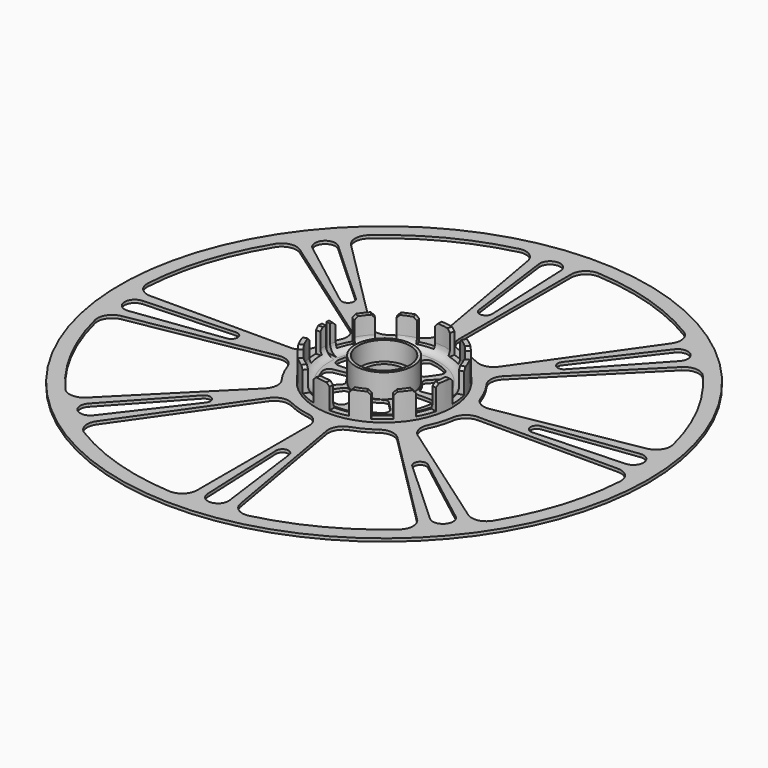
from build123d import *

# Parameters (mm, degrees)
F0_R      = 89
F0_R_2    = 6.5
F1_DEPTH  = 1
F2_R      = 23
F2_R_2    = 21.5
F3_DEPTH  = 9
F4_R      = 3
F6_DEPTH  = 1
F7_R      = 8
F7_R_2    = 6.5
F8_DEPTH  = 2
F9_R      = 9.75
F9_R_2    = 8.75
F10_DEPTH = 8
F12_DEPTH = 8
F15_DEPTH = 9
F16_SIZE  = 1


# Not quite as in the source:
# - a fillet or chamfer that OpenCascade refuses, or shapes differently, is made with other operations: its cross-section is extruded or revolved along the edge and cut away or added


with BuildPart() as f1:
    # F0 (on Top) → F1 (new body)
    with BuildSketch(Plane.XY):
        Circle(F0_R)
        Circle(F0_R_2, mode=Mode.SUBTRACT)
    extrude(amount=F1_DEPTH)

    # F2 (on face) → F3 (join)
    with BuildSketch(Plane.XY.offset(1)):
        Circle(F2_R)
        Circle(F2_R_2, mode=Mode.SUBTRACT)
    extrude(amount=F3_DEPTH)

    # F4
    f4_edges = [f1.edges().sort_by_distance(p)[0] for p in [
        (-21.5, 0, 1),
    ]]
    fillet(f4_edges, radius=F4_R)

    # F5 (on face) → F6 (cut, through all)
    with BuildSketch(Plane.XY.offset(1)):
        with BuildLine():
            ThreePointArc((-83.8315889079, 5.3164556962), (-82.4873148521, 1.5781787365), (-78.8416133777, 0))
            Line((-78.8416133777, 0), (-31.6069612586, 0))
            ThreePointArc((-31.6069612586, 0), (-28.3593659944, 1.1982734186), (-26.6683735619, 4.21875))
            ThreePointArc((-26.6683735619, 4.21875), (-25.7503576702, 8.1190565866), (-24.265228312, 11.8405529841))
            ThreePointArc((-24.265228312, 11.8405529841), (-23.9179340262, 15.2846959638), (-25.8909069287, 18.1290082026))
            Line((-25.8909069287, 18.1290082026), (-64.5832687734, 45.2216916374))
            ThreePointArc((-64.5832687734, 45.2216916374), (-68.4748587246, 46.0200117588), (-71.7202111422, 43.7288384675))
            ThreePointArc((-71.7202111422, 43.7288384675), (-80.1122238629, 25.2592871584), (-83.8315889079, 5.3164556962))
        make_face()
        with BuildLine():
            ThreePointArc((-81.6348058606, -19.792889433), (-74.508909987, -38.7868835117), (-63.0371868691, -55.5185831198))
            ThreePointArc((-63.0371868691, -55.5185831198), (-59.4432805803, -57.2113988073), (-55.7494394591, -55.7494394591))
            Line((-55.7494394591, -55.7494394591), (-22.3494966386, -22.3494966386))
            ThreePointArc((-22.3494966386, -22.3494966386), (-20.9004072647, -19.2057927448), (-21.840494522, -15.8742810557))
            ThreePointArc((-21.840494522, -15.8742810557), (-23.9492924958, -12.4672125573), (-25.5306427945, -8.7855721784))
            ThreePointArc((-25.5306427945, -8.7855721784), (-27.7204455063, -6.1046211775), (-31.1267804966, -5.4884912241))
            Line((-31.1267804966, -5.4884912241), (-77.6438321144, -13.6907024874))
            ThreePointArc((-77.6438321144, -13.6907024874), (-80.9600993299, -15.87797456), (-81.6348058606, -19.792889433))
        make_face()
        with BuildLine():
            ThreePointArc((-43.7288384675, -71.7202111422), (-25.2592871584, -80.1122238629), (-5.3164556962, -83.8315889079))
            ThreePointArc((-5.3164556962, -83.8315889079), (-1.5781787365, -82.4873148521), (0, -78.8416133777))
            Line((0, -78.8416133777), (0, -31.6069612586))
            ThreePointArc((0, -31.6069612586), (-1.1982734186, -28.3593659944), (-4.21875, -26.6683735619))
            ThreePointArc((-4.21875, -26.6683735619), (-8.1190565866, -25.7503576702), (-11.8405529841, -24.265228312))
            ThreePointArc((-11.8405529841, -24.265228312), (-15.2846959638, -23.9179340262), (-18.1290082026, -25.8909069287))
            Line((-18.1290082026, -25.8909069287), (-45.2216916374, -64.5832687734))
            ThreePointArc((-45.2216916374, -64.5832687734), (-46.0200117588, -68.4748587246), (-43.7288384675, -71.7202111422))
        make_face()
        with BuildLine():
            ThreePointArc((19.792889433, -81.6348058606), (38.7868835117, -74.508909987), (55.5185831198, -63.0371868691))
            ThreePointArc((55.5185831198, -63.0371868691), (57.2113988073, -59.4432805803), (55.7494394591, -55.7494394591))
            Line((55.7494394591, -55.7494394591), (22.3494966386, -22.3494966386))
            ThreePointArc((22.3494966386, -22.3494966386), (19.2057927448, -20.9004072647), (15.8742810557, -21.840494522))
            ThreePointArc((15.8742810557, -21.840494522), (12.4672125573, -23.9492924958), (8.7855721784, -25.5306427945))
            ThreePointArc((8.7855721784, -25.5306427945), (6.1046211775, -27.7204455063), (5.4884912241, -31.1267804966))
            Line((5.4884912241, -31.1267804966), (13.6907024874, -77.6438321144))
            ThreePointArc((13.6907024874, -77.6438321144), (15.87797456, -80.9600993299), (19.792889433, -81.6348058606))
        make_face()
        with BuildLine():
            ThreePointArc((71.7202111422, -43.7288384675), (80.1122238629, -25.2592871584), (83.8315889079, -5.3164556962))
            ThreePointArc((83.8315889079, -5.3164556962), (82.4873148521, -1.5781787365), (78.8416133777, 0))
            Line((78.8416133777, 0), (31.6069612586, 0))
            ThreePointArc((31.6069612586, 0), (28.3593659944, -1.1982734186), (26.6683735619, -4.21875))
            ThreePointArc((26.6683735619, -4.21875), (25.7503576702, -8.1190565866), (24.265228312, -11.8405529841))
            ThreePointArc((24.265228312, -11.8405529841), (23.9179340262, -15.2846959638), (25.8909069287, -18.1290082026))
            Line((25.8909069287, -18.1290082026), (64.5832687734, -45.2216916374))
            ThreePointArc((64.5832687734, -45.2216916374), (68.4748587246, -46.0200117588), (71.7202111422, -43.7288384675))
        make_face()
        with BuildLine():
            ThreePointArc((81.6348058606, 19.792889433), (74.508909987, 38.7868835117), (63.0371868691, 55.5185831198))
            ThreePointArc((63.0371868691, 55.5185831198), (59.4432805803, 57.2113988073), (55.7494394591, 55.7494394591))
            Line((55.7494394591, 55.7494394591), (22.3494966386, 22.3494966386))
            ThreePointArc((22.3494966386, 22.3494966386), (20.9004072647, 19.2057927448), (21.840494522, 15.8742810557))
            ThreePointArc((21.840494522, 15.8742810557), (23.9492924958, 12.4672125573), (25.5306427945, 8.7855721784))
            ThreePointArc((25.5306427945, 8.7855721784), (27.7204455063, 6.1046211775), (31.1267804966, 5.4884912241))
            Line((31.1267804966, 5.4884912241), (77.6438321144, 13.6907024874))
            ThreePointArc((77.6438321144, 13.6907024874), (80.9600993299, 15.87797456), (81.6348058606, 19.792889433))
        make_face()
        with BuildLine():
            ThreePointArc((43.7288384675, 71.7202111422), (25.2592871584, 80.1122238629), (5.3164556962, 83.8315889079))
            ThreePointArc((5.3164556962, 83.8315889079), (1.5781787365, 82.4873148521), (0, 78.8416133777))
            Line((0, 78.8416133777), (0, 31.6069612586))
            ThreePointArc((0, 31.6069612586), (1.1982734186, 28.3593659944), (4.21875, 26.6683735619))
            ThreePointArc((4.21875, 26.6683735619), (8.1190565866, 25.7503576702), (11.8405529841, 24.265228312))
            ThreePointArc((11.8405529841, 24.265228312), (15.2846959638, 23.9179340262), (18.1290082026, 25.8909069287))
            Line((18.1290082026, 25.8909069287), (45.2216916374, 64.5832687734))
            ThreePointArc((45.2216916374, 64.5832687734), (46.0200117588, 68.4748587246), (43.7288384675, 71.7202111422))
        make_face()
        with BuildLine():
            ThreePointArc((-19.792889433, 81.6348058606), (-38.7868835117, 74.508909987), (-55.5185831198, 63.0371868691))
            ThreePointArc((-55.5185831198, 63.0371868691), (-57.2113988073, 59.4432805803), (-55.7494394591, 55.7494394591))
            Line((-55.7494394591, 55.7494394591), (-22.3494966386, 22.3494966386))
            ThreePointArc((-22.3494966386, 22.3494966386), (-19.2057927448, 20.9004072647), (-15.8742810557, 21.840494522))
            ThreePointArc((-15.8742810557, 21.840494522), (-12.4672125573, 23.9492924958), (-8.7855721784, 25.5306427945))
            ThreePointArc((-8.7855721784, 25.5306427945), (-6.1046211775, 27.7204455063), (-5.4884912241, 31.1267804966))
            Line((-5.4884912241, 31.1267804966), (-13.6907024874, 77.6438321144))
            ThreePointArc((-13.6907024874, 77.6438321144), (-15.87797456, 80.9600993299), (-19.792889433, 81.6348058606))
        make_face()
        with BuildLine():
            ThreePointArc((-17.3537069424, 2.2580645161), (-16.8731119165, 0.6801759648), (-15.3704261489, 0))
            Line((-15.3704261489, 0), (-11.401754251, 0))
            ThreePointArc((-11.401754251, 0), (-10.4126835409, 0.3722858827), (-9.9145689139, 1.3043478261))
            ThreePointArc((-9.9145689139, 1.3043478261), (-9.5371695075, 3.007057995), (-8.8696825719, 4.6183039174))
            ThreePointArc((-8.8696825719, 4.6183039174), (-8.7431054189, 5.6675111764), (-9.3397703032, 6.5397775714))
            Line((-9.3397703032, 6.5397775714), (-12.5907160015, 8.8161142557))
            ThreePointArc((-12.5907160015, 8.8161142557), (-14.2117770259, 9.1208518712), (-15.510497116, 8.103979221))
            ThreePointArc((-15.510497116, 8.103979221), (-16.6900466381, 5.2623514913), (-17.3537069424, 2.2580645161))
        make_face()
        with BuildLine():
            ThreePointArc((-16.697956352, -5.2371990286), (-15.5226895806, -8.0806007316), (-13.8676165894, -10.6742311259))
            ThreePointArc((-13.8676165894, -10.6742311259), (-12.412048893, -11.4501348188), (-10.8685325596, -10.8685325596))
            Line((-10.8685325596, -10.8685325596), (-8.0622577483, -8.0622577483))
            ThreePointArc((-8.0622577483, -8.0622577483), (-7.6261250143, -7.0996332699), (-7.9329721044, -6.0883457187))
            ThreePointArc((-7.9329721044, -6.0883457187), (-8.8701083318, -4.6174861324), (-9.5374467111, -3.006178676))
            ThreePointArc((-9.5374467111, -3.006178676), (-10.1898447156, -2.1747735451), (-11.2285359843, -1.9798938479))
            Line((-11.2285359843, -1.9798938479), (-15.1369148386, -2.6690464907))
            ThreePointArc((-15.1369148386, -2.6690464907), (-16.4986601161, -3.5998276994), (-16.697956352, -5.2371990286))
        make_face()
        with BuildLine():
            ThreePointArc((-8.103979221, -15.510497116), (-5.2623514913, -16.6900466381), (-2.2580645161, -17.3537069424))
            ThreePointArc((-2.2580645161, -17.3537069424), (-0.6801759648, -16.8731119165), (0, -15.3704261489))
            Line((0, -15.3704261489), (0, -11.401754251))
            ThreePointArc((0, -11.401754251), (-0.3722858827, -10.4126835409), (-1.3043478261, -9.9145689139))
            ThreePointArc((-1.3043478261, -9.9145689139), (-3.007057995, -9.5371695075), (-4.6183039174, -8.8696825719))
            ThreePointArc((-4.6183039174, -8.8696825719), (-5.6675111764, -8.7431054189), (-6.5397775714, -9.3397703032))
            Line((-6.5397775714, -9.3397703032), (-8.8161142557, -12.5907160015))
            ThreePointArc((-8.8161142557, -12.5907160015), (-9.1208518712, -14.2117770259), (-8.103979221, -15.510497116))
        make_face()
        with BuildLine():
            ThreePointArc((5.2371990286, -16.697956352), (8.0806007316, -15.5226895806), (10.6742311259, -13.8676165894))
            ThreePointArc((10.6742311259, -13.8676165894), (11.4501348188, -12.412048893), (10.8685325596, -10.8685325596))
            Line((10.8685325596, -10.8685325596), (8.0622577483, -8.0622577483))
            ThreePointArc((8.0622577483, -8.0622577483), (7.0996332699, -7.6261250143), (6.0883457187, -7.9329721044))
            ThreePointArc((6.0883457187, -7.9329721044), (4.6174861324, -8.8701083318), (3.006178676, -9.5374467111))
            ThreePointArc((3.006178676, -9.5374467111), (2.1747735451, -10.1898447156), (1.9798938479, -11.2285359843))
            Line((1.9798938479, -11.2285359843), (2.6690464907, -15.1369148386))
            ThreePointArc((2.6690464907, -15.1369148386), (3.5998276994, -16.4986601161), (5.2371990286, -16.697956352))
        make_face()
        with BuildLine():
            ThreePointArc((15.510497116, -8.103979221), (16.6900466381, -5.2623514913), (17.3537069424, -2.2580645161))
            ThreePointArc((17.3537069424, -2.2580645161), (16.8731119165, -0.6801759648), (15.3704261489, 0))
            Line((15.3704261489, 0), (11.401754251, 0))
            ThreePointArc((11.401754251, 0), (10.4126835409, -0.3722858827), (9.9145689139, -1.3043478261))
            ThreePointArc((9.9145689139, -1.3043478261), (9.5371695075, -3.007057995), (8.8696825719, -4.6183039174))
            ThreePointArc((8.8696825719, -4.6183039174), (8.7431054189, -5.6675111764), (9.3397703032, -6.5397775714))
            Line((9.3397703032, -6.5397775714), (12.5907160015, -8.8161142557))
            ThreePointArc((12.5907160015, -8.8161142557), (14.2117770259, -9.1208518712), (15.510497116, -8.103979221))
        make_face()
        with BuildLine():
            ThreePointArc((16.697956352, 5.2371990286), (15.5226895806, 8.0806007316), (13.8676165894, 10.6742311259))
            ThreePointArc((13.8676165894, 10.6742311259), (12.412048893, 11.4501348188), (10.8685325596, 10.8685325596))
            Line((10.8685325596, 10.8685325596), (8.0622577483, 8.0622577483))
            ThreePointArc((8.0622577483, 8.0622577483), (7.6261250143, 7.0996332699), (7.9329721044, 6.0883457187))
            ThreePointArc((7.9329721044, 6.0883457187), (8.8701083318, 4.6174861324), (9.5374467111, 3.006178676))
            ThreePointArc((9.5374467111, 3.006178676), (10.1898447156, 2.1747735451), (11.2285359843, 1.9798938479))
            Line((11.2285359843, 1.9798938479), (15.1369148386, 2.6690464907))
            ThreePointArc((15.1369148386, 2.6690464907), (16.4986601161, 3.5998276994), (16.697956352, 5.2371990286))
        make_face()
        with BuildLine():
            ThreePointArc((8.103979221, 15.510497116), (5.2623514913, 16.6900466381), (2.2580645161, 17.3537069424))
            ThreePointArc((2.2580645161, 17.3537069424), (0.6801759648, 16.8731119165), (0, 15.3704261489))
            Line((0, 15.3704261489), (0, 11.401754251))
            ThreePointArc((0, 11.401754251), (0.3722858827, 10.4126835409), (1.3043478261, 9.9145689139))
            ThreePointArc((1.3043478261, 9.9145689139), (3.007057995, 9.5371695075), (4.6183039174, 8.8696825719))
            ThreePointArc((4.6183039174, 8.8696825719), (5.6675111764, 8.7431054189), (6.5397775714, 9.3397703032))
            Line((6.5397775714, 9.3397703032), (8.8161142557, 12.5907160015))
            ThreePointArc((8.8161142557, 12.5907160015), (9.1208518712, 14.2117770259), (8.103979221, 15.510497116))
        make_face()
        with BuildLine():
            ThreePointArc((-5.2371990286, 16.697956352), (-8.0806007316, 15.5226895806), (-10.6742311259, 13.8676165894))
            ThreePointArc((-10.6742311259, 13.8676165894), (-11.4501348188, 12.412048893), (-10.8685325596, 10.8685325596))
            Line((-10.8685325596, 10.8685325596), (-8.0622577483, 8.0622577483))
            ThreePointArc((-8.0622577483, 8.0622577483), (-7.0996332699, 7.6261250143), (-6.0883457187, 7.9329721044))
            ThreePointArc((-6.0883457187, 7.9329721044), (-4.6174861324, 8.8701083318), (-3.006178676, 9.5374467111))
            ThreePointArc((-3.006178676, 9.5374467111), (-2.1747735451, 10.1898447156), (-1.9798938479, 11.2285359843))
            Line((-1.9798938479, 11.2285359843), (-2.6690464907, 15.1369148386))
            ThreePointArc((-2.6690464907, 15.1369148386), (-3.5998276994, 16.4986601161), (-5.2371990286, 16.697956352))
        make_face()
        with BuildLine():
            ThreePointArc((-58.0728096368, 53.213925833), (-63.0306241772, 52.8889735), (-62.489724294, 47.9500519221))
            Line((-62.489724294, 47.9500519221), (-38.3032770261, 29.3911381902))
            ThreePointArc((-38.3032770261, 29.3911381902), (-35.4052410939, 29.7085247437), (-35.5959150138, 32.6176465948))
            Line((-35.5959150138, 32.6176465948), (-58.0728096368, 53.213925833))
        make_face()
        with BuildLine():
            Line((-78.0927146751, -10.2811009304), (-47.8671800479, -6.3018338058))
            ThreePointArc((-47.8671800479, -6.3018338058), (-46.0423853723, -4.0281867618), (-48.2342719823, -2.1059537953))
            Line((-48.2342719823, -2.1059537953), (-78.6916053068, -3.4357496867))
            ThreePointArc((-78.6916053068, -3.4357496867), (-81.96753359, -7.1712299663), (-78.0927146751, -10.2811009304))
        make_face()
        with BuildLine():
            Line((-47.9500519221, -62.489724294), (-29.3911381902, -38.3032770261))
            ThreePointArc((-29.3911381902, -38.3032770261), (-29.7085247437, -35.4052410939), (-32.6176465948, -35.5959150138))
            Line((-32.6176465948, -35.5959150138), (-53.213925833, -58.0728096368))
            ThreePointArc((-53.213925833, -58.0728096368), (-52.8889735, -63.0306241772), (-47.9500519221, -62.489724294))
        make_face()
        with BuildLine():
            Line((10.2811009304, -78.0927146751), (6.3018338058, -47.8671800479))
            ThreePointArc((6.3018338058, -47.8671800479), (4.0281867618, -46.0423853723), (2.1059537953, -48.2342719823))
            Line((2.1059537953, -48.2342719823), (3.4357496867, -78.6916053068))
            ThreePointArc((3.4357496867, -78.6916053068), (7.1712299663, -81.96753359), (10.2811009304, -78.0927146751))
        make_face()
        with BuildLine():
            Line((62.489724294, -47.9500519221), (38.3032770261, -29.3911381902))
            ThreePointArc((38.3032770261, -29.3911381902), (35.4052410939, -29.7085247437), (35.5959150138, -32.6176465948))
            Line((35.5959150138, -32.6176465948), (58.0728096368, -53.213925833))
            ThreePointArc((58.0728096368, -53.213925833), (63.0306241772, -52.8889735), (62.489724294, -47.9500519221))
        make_face()
        with BuildLine():
            Line((78.0927146751, 10.2811009304), (47.8671800479, 6.3018338058))
            ThreePointArc((47.8671800479, 6.3018338058), (46.0423853723, 4.0281867618), (48.2342719823, 2.1059537953))
            Line((48.2342719823, 2.1059537953), (78.6916053068, 3.4357496867))
            ThreePointArc((78.6916053068, 3.4357496867), (81.96753359, 7.1712299663), (78.0927146751, 10.2811009304))
        make_face()
        with BuildLine():
            Line((47.9500519221, 62.489724294), (29.3911381902, 38.3032770261))
            ThreePointArc((29.3911381902, 38.3032770261), (29.7085247437, 35.4052410939), (32.6176465948, 35.5959150138))
            Line((32.6176465948, 35.5959150138), (53.213925833, 58.0728096368))
            ThreePointArc((53.213925833, 58.0728096368), (52.8889735, 63.0306241772), (47.9500519221, 62.489724294))
        make_face()
        with BuildLine():
            Line((-10.2811009304, 78.0927146751), (-6.3018338058, 47.8671800479))
            ThreePointArc((-6.3018338058, 47.8671800479), (-4.0281867618, 46.0423853723), (-2.1059537953, 48.2342719823))
            Line((-2.1059537953, 48.2342719823), (-3.4357496867, 78.6916053068))
            ThreePointArc((-3.4357496867, 78.6916053068), (-7.1712299663, 81.96753359), (-10.2811009304, 78.0927146751))
        make_face()
    extrude(amount=-F6_DEPTH, mode=Mode.SUBTRACT)

    # F7 (on face) → F8 (join)
    with BuildSketch(Plane.XY.offset(1)):
        Circle(F7_R)
        Circle(F7_R_2, mode=Mode.SUBTRACT)
    extrude(amount=F8_DEPTH)

    # F9 (on face) → F10 (join)
    with BuildSketch(Plane.XY.offset(1)):
        Circle(F9_R)
        Circle(F9_R_2, mode=Mode.SUBTRACT)
    extrude(amount=F10_DEPTH)

    # F11 (on face) → F12 (cut)
    with BuildSketch(Plane.XY.offset(10)):
        with BuildLine():
            ThreePointArc((-20.7846096908, 12), (-22.1731087803, 9.1844023768), (-23.1822198309, 6.2116570825))
            Line((-23.1822198309, 6.2116570825), (-20.2844423521, 5.4351999472))
            ThreePointArc((-20.2844423521, 5.4351999472), (-19.4014701827, 8.0363520797), (-18.1865334795, 10.5))
            Line((-18.1865334795, 10.5), (-20.7846096908, 12))
        make_face()
        with BuildLine():
            ThreePointArc((-24, 0), (-23.794676673, -3.1326286133), (-23.1822198309, -6.2116570825))
            Line((-23.1822198309, -6.2116570825), (-20.2844423521, -5.4351999472))
            ThreePointArc((-20.2844423521, -5.4351999472), (-20.8203420889, -2.7410500366), (-21, 0))
            Line((-21, 0), (-24, 0))
        make_face()
        with BuildLine():
            ThreePointArc((-20.7846096908, -12), (-19.040480167, -14.6102742962), (-16.9705627485, -16.9705627485))
            Line((-16.9705627485, -16.9705627485), (-14.8492424049, -14.8492424049))
            ThreePointArc((-14.8492424049, -14.8492424049), (-16.6604201461, -12.7839900092), (-18.1865334795, -10.5))
            Line((-18.1865334795, -10.5), (-20.7846096908, -12))
        make_face()
        with BuildLine():
            ThreePointArc((-12, -20.7846096908), (-9.1844023768, -22.1731087803), (-6.2116570825, -23.1822198309))
            Line((-6.2116570825, -23.1822198309), (-5.4351999472, -20.2844423521))
            ThreePointArc((-5.4351999472, -20.2844423521), (-8.0363520797, -19.4014701827), (-10.5, -18.1865334795))
            Line((-10.5, -18.1865334795), (-12, -20.7846096908))
        make_face()
        with BuildLine():
            ThreePointArc((0, -24), (3.1326286133, -23.794676673), (6.2116570825, -23.1822198309))
            Line((6.2116570825, -23.1822198309), (5.4351999472, -20.2844423521))
            ThreePointArc((5.4351999472, -20.2844423521), (2.7410500366, -20.8203420889), (0, -21))
            Line((0, -21), (0, -24))
        make_face()
        with BuildLine():
            ThreePointArc((12, -20.7846096908), (14.6102742962, -19.040480167), (16.9705627485, -16.9705627485))
            Line((16.9705627485, -16.9705627485), (14.8492424049, -14.8492424049))
            ThreePointArc((14.8492424049, -14.8492424049), (12.7839900092, -16.6604201461), (10.5, -18.1865334795))
            Line((10.5, -18.1865334795), (12, -20.7846096908))
        make_face()
        with BuildLine():
            ThreePointArc((20.7846096908, -12), (22.1731087803, -9.1844023768), (23.1822198309, -6.2116570825))
            Line((23.1822198309, -6.2116570825), (20.2844423521, -5.4351999472))
            ThreePointArc((20.2844423521, -5.4351999472), (19.4014701827, -8.0363520797), (18.1865334795, -10.5))
            Line((18.1865334795, -10.5), (20.7846096908, -12))
        make_face()
        with BuildLine():
            ThreePointArc((24, 0), (23.794676673, 3.1326286133), (23.1822198309, 6.2116570825))
            Line((23.1822198309, 6.2116570825), (20.2844423521, 5.4351999472))
            ThreePointArc((20.2844423521, 5.4351999472), (20.8203420889, 2.7410500366), (21, 0))
            Line((21, 0), (24, 0))
        make_face()
        with BuildLine():
            ThreePointArc((20.7846096908, 12), (19.040480167, 14.6102742962), (16.9705627485, 16.9705627485))
            Line((16.9705627485, 16.9705627485), (14.8492424049, 14.8492424049))
            ThreePointArc((14.8492424049, 14.8492424049), (16.6604201461, 12.7839900092), (18.1865334795, 10.5))
            Line((18.1865334795, 10.5), (20.7846096908, 12))
        make_face()
        with BuildLine():
            ThreePointArc((12, 20.7846096908), (9.1844023768, 22.1731087803), (6.2116570825, 23.1822198309))
            Line((6.2116570825, 23.1822198309), (5.4351999472, 20.2844423521))
            ThreePointArc((5.4351999472, 20.2844423521), (8.0363520797, 19.4014701827), (10.5, 18.1865334795))
            Line((10.5, 18.1865334795), (12, 20.7846096908))
        make_face()
        with BuildLine():
            ThreePointArc((0, 24), (-3.1326286133, 23.794676673), (-6.2116570825, 23.1822198309))
            Line((-6.2116570825, 23.1822198309), (-5.4351999472, 20.2844423521))
            ThreePointArc((-5.4351999472, 20.2844423521), (-2.7410500366, 20.8203420889), (0, 21))
            Line((0, 21), (0, 24))
        make_face()
        with BuildLine():
            ThreePointArc((-12, 20.7846096908), (-14.6102742962, 19.040480167), (-16.9705627485, 16.9705627485))
            Line((-16.9705627485, 16.9705627485), (-14.8492424049, 14.8492424049))
            ThreePointArc((-14.8492424049, 14.8492424049), (-12.7839900092, 16.6604201461), (-10.5, 18.1865334795))
            Line((-10.5, 18.1865334795), (-12, 20.7846096908))
        make_face()
    extrude(amount=-F12_DEPTH, mode=Mode.SUBTRACT)

    # F13: fillet of radius 1 on 1 edges, made by hand

    # F13_s1 → F13_t2 (revolve)
    with BuildSketch(Plane.XZ):
        with BuildLine():
            ThreePointArc((8.75, 1.9682458366), (8.540569415, 1.3558734009), (8, 1))
            Line((8, 1), (8.75, 1))
            Line((8.75, 1), (8.75, 1.9682458366))
        make_face()
    revolve(axis=Axis((0, 0, 1), (0, 0, 1)))

    # F14 (on face) → F15 (cut, through all)
    with BuildSketch(Plane.XY.offset(10)):
        Polygon((-23.6690532746, 4.1734927001), (-23.8685254888, 2.5086831184), (-13.9233065352, 1.4633984857), (-13.8209757444, 2.4370109235), align=None)
    extrude(amount=-F15_DEPTH, mode=Mode.SUBTRACT)

    # F16
    f16_edges = [f1.edges().sort_by_distance(p)[0] for p in [
        (-11.125, 19.269065, 10),
        (-5.758724, 21.49185, 10),
        (0, 22.25, 10),
        (5.758724, 21.49185, 10),
        (11.125, 19.269065, 10),
        (15.733126, 15.733126, 10),
        (-15.733126, 15.733126, 10),
        (-19.269065, 11.125, 10),
        (-21.49185, 5.758724, 10),
        (-22.25, 0, 10),
        (-21.49185, -5.758724, 10),
        (-19.269065, -11.125, 10),
        (-15.733126, -15.733126, 10),
        (-11.125, -19.269065, 10),
        (-5.758724, -21.49185, 10),
        (0, -22.25, 10),
        (5.758724, -21.49185, 10),
        (11.125, -19.269065, 10),
        (15.733126, -15.733126, 10),
        (19.269065, -11.125, 10),
        (21.49185, -5.758724, 10),
        (22.25, 0, 10),
        (21.49185, 5.758724, 10),
        (19.269065, 11.125, 10),
    ]]
    chamfer(f16_edges, length=F16_SIZE)


solid = f1.part
